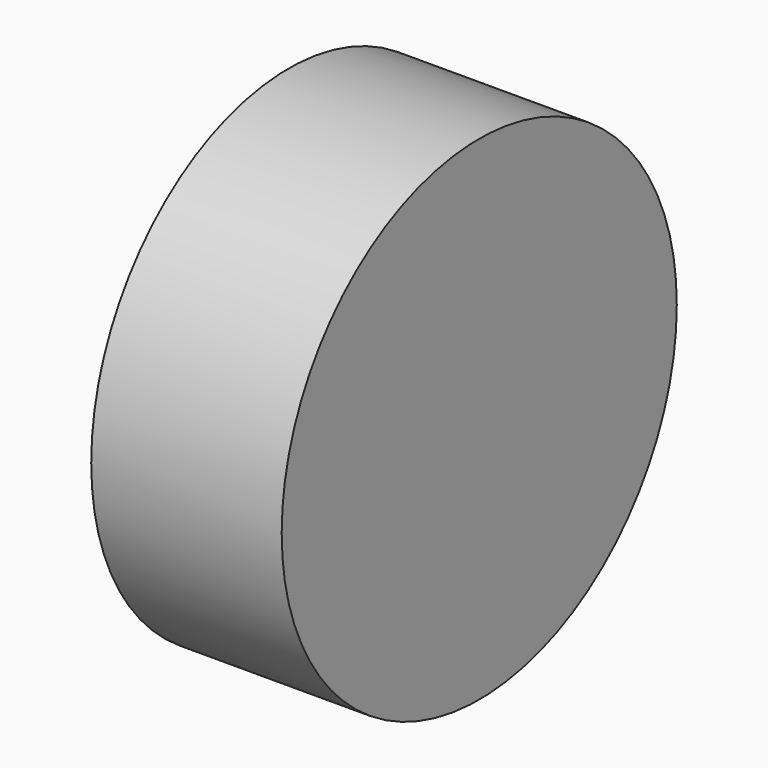
from build123d import *

# Parameters (mm, degrees)
F0_W = 67.9279565811
F0_H = 88.0647003651


# Not quite as in the source:
# - a feature of the source that left no trace in its solid (it failed there, or was rolled back) is left out


with BuildPart() as f1:
    # F0 (on Top) → F1 (revolve)
    with BuildSketch(Plane.XY):
        Rectangle(F0_W, F0_H)
    revolve(axis=Axis((0, 44.0323501825, 0), (-1, 0, 0)))


solid = f1.part
